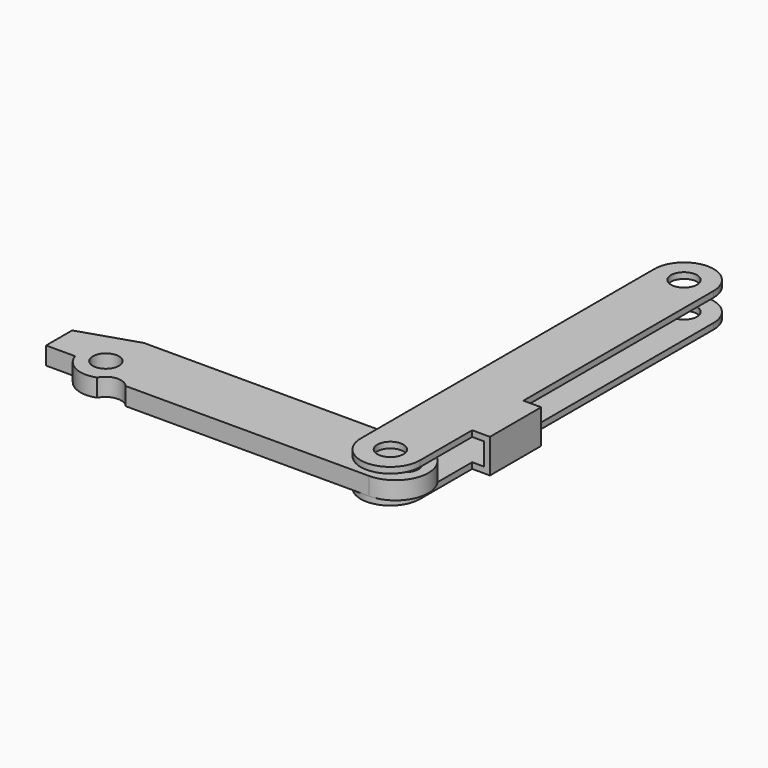
from build123d import *

# Parameters (mm, degrees)
F0_R     = 2.2
F1_DEPTH = 3.75
F2_T     = 1
F3_R     = 2.2
F4_DEPTH = 3


with BuildPart() as f1:
    # F0 (on Top) → F1 (new body)
    with BuildSketch(Plane.XY):
        with BuildLine():
            Line((-5, 50.93), (-5, 0))
            Line((-5, 0), (-5, -11))
            ThreePointArc((-5, -11), (0, -16), (5, -11))
            Line((5, -11), (5, 0))
            Line((5, 0), (7, 0))
            Line((7, 0), (7, 10.8))
            Line((7, 10.8), (5, 10.8))
            Line((5, 10.8), (5, 50.93))
            ThreePointArc((5, 50.93), (0, 55.93), (-5, 50.93))
        make_face()
        with Locations((0, -11)):
            Circle(F0_R, mode=Mode.SUBTRACT)
        with Locations((0, 50.93)):
            Circle(F0_R, mode=Mode.SUBTRACT)
    extrude(amount=F1_DEPTH)

    # F2
    f2_openings = [f1.faces().sort_by_distance(p)[0] for p in [
        (-5, 19.965, 1.875),
        (0, 55.93, 1.875),
        (0, -16, 1.875),
        (5, -5.5, 1.875),
        (6, 0, 1.875),
        (6, 10.8, 1.875),
        (5, 30.865, 1.875),
        (-2.2, 50.93, 1.875),
        (-2.2, -11, 1.875),
    ]]
    offset(amount=F2_T, openings=f2_openings, kind=Kind.INTERSECTION)


with BuildPart() as f4:
    # F3 (on Top) → F4 (new body)
    with BuildSketch(Plane.XY):
        with BuildLine():
            Line((0.4625649198, -4.9407491021), (-46.4374350802, -4.9407491021))
            Line((-46.4374350802, -4.9407491021), (-56.0463459179, -8.0518313113))
            Line((-56.0463459179, -8.0518313113), (-56.0463459179, -13.5518313113))
            Line((-56.0463459179, -13.5518313113), (-51.1463459179, -13.5518313113))
            ThreePointArc((-51.1463459179, -13.5518313113), (-48.7478397903, -16.3395991716), (-45.0740717351, -16.5066607296))
            ThreePointArc((-45.0740717351, -16.5066607296), (-42.9811130235, -15.0799698083), (-40.6374350802, -16.0407491021))
            Line((-40.6374350802, -16.0407491021), (0.4625649198, -16.0407491021))
            ThreePointArc((0.4625649198, -16.0407491021), (6.0125649198, -10.4907491021), (0.4625649198, -4.9407491021))
        make_face()
        with Locations((-47.1068173292, -12.1095654204)):
            Circle(F3_R, mode=Mode.SUBTRACT)
        with Locations((2.1364323051, -10.4907491021)):
            Circle(F3_R, mode=Mode.SUBTRACT)
    extrude(amount=F4_DEPTH)


solid = Compound([f1.part, f4.part])
